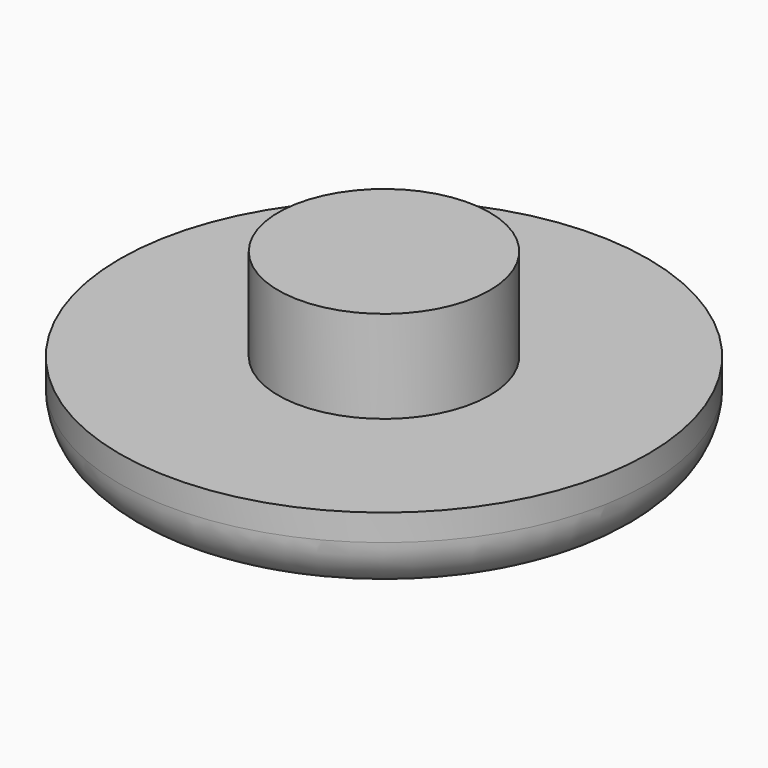
from build123d import *

# Parameters (mm, degrees)
F0_R         = 10
F1_DEPTH     = 3
F2_R         = 4
F3_DEPTH     = 3.5
F4_R         = 2
F5_TEXT_SIZE = 9.233432721
F6_DEPTH     = 1.5


# Not quite as in the source:
# - Text() gives the source's letters only with a copy of the font that has no kerning and outlines rounded to 1/6400 em; it was checked with that copy


with BuildPart() as f1:
    # F0 (on Top) → F1 (new body)
    with BuildSketch(Plane.XY):
        Circle(F0_R)
    extrude(amount=F1_DEPTH)

    # F2 (on face) → F3 (join)
    with BuildSketch(Plane.XY.offset(3)):
        Circle(F2_R)
    extrude(amount=F3_DEPTH)

    # F4
    f4_edges = [f1.edges().sort_by_distance(p)[0] for p in [
        (-10, 0, 0),
    ]]
    fillet(f4_edges, radius=F4_R)

    # F5 (on face) → F6 (cut)
    with BuildSketch(Plane(origin=(0, 0, 0), x_dir=(1, 0, 0), z_dir=(0, 0, -1))):
        with Locations((-7.8558754234, -3.5792409305)):
            Text('CM', F5_TEXT_SIZE, font='Arimo', font_style=FontStyle.ITALIC, text_align=(TextAlign.LEFT, TextAlign.BOTTOM))
    extrude(amount=-F6_DEPTH, mode=Mode.SUBTRACT)


solid = f1.part
